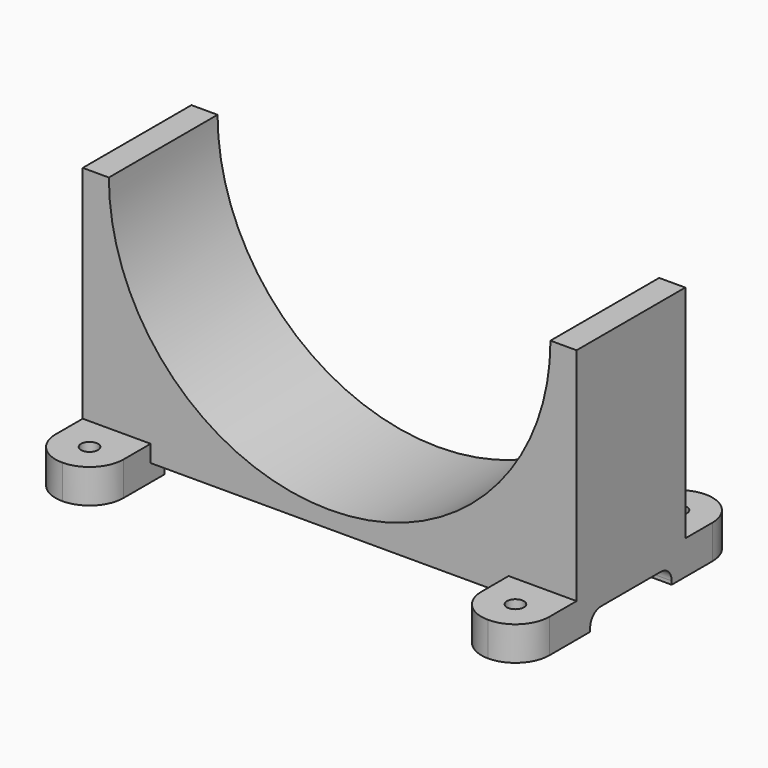
from build123d import *

# Parameters (mm, degrees)
F1_DEPTH      = 25.4
F2_W          = 12.7
F2_H          = 6.35
F3_DEPTH      = 12.7
F3_DEPTH_BACK = 38.1
F4_R          = 6.34999
F5_W          = 19.05
F5_H          = 3.175
F6_DEPTH      = 92.3136190901
F7_W          = 66.9126190901
F7_H          = 3.175
F8_DEPTH      = 38.101
F9_R          = 2.54
F10_R         = 1.5875
F11_DEPTH     = 6.351


# Not quite as in the source:
# - a fillet or chamfer is up to 0.001 mm smaller than in the source, because OpenCascade refuses the exact size


with BuildPart() as f1:
    # F0 (on Front) → F1 (new body)
    with BuildSketch(Plane.XZ):
        with BuildLine():
            ThreePointArc((41.275, 0), (0, -41.275), (-41.275, 0))
            Line((-41.275, 0), (-46.156309545, 0))
            Line((-46.156309545, 0), (-46.156309545, -47.625))
            Line((-46.156309545, -47.625), (46.156309545, -47.625))
            Line((46.156309545, -47.625), (46.156309545, 0))
            Line((46.156309545, 0), (41.275, 0))
        make_face()
    extrude(amount=F1_DEPTH)

    # F2 (on face) → F3 (join, two sides)
    with BuildSketch(Plane.XZ.offset(25.4)) as f3_sk:
        with Locations((-39.806309545, -44.45)):
            Rectangle(F2_W, F2_H)
        with Locations((39.806309545, -44.45)):
            Rectangle(F2_W, F2_H)
    extrude(amount=F3_DEPTH)
    extrude(f3_sk.sketch, amount=-F3_DEPTH_BACK)

    # F4 (radius 6.35 in the source; OpenCascade refuses exactly that, so slightly less here)
    f4_edges = [f1.edges().sort_by_distance(p)[0] for p in [
        (-46.15631, 12.7, -44.45),
        (-33.45631, 12.7, -44.45),
        (-46.15631, -38.1, -44.45),
        (-33.45631, -38.1, -44.45),
        (33.45631, -38.1, -44.45),
        (46.15631, -38.1, -44.45),
        (33.45631, 12.7, -44.45),
        (46.15631, 12.7, -44.45),
    ]]
    fillet(f4_edges, radius=F4_R)

    # F5 (on face) → F6 (cut, through all)
    with BuildSketch(Plane(origin=(-46.156309545, 0, 0), x_dir=(0, -1, 0), z_dir=(-1, 0, 0))):
        with Locations((12.7, -46.0375)):
            Rectangle(F5_W, F5_H)
    extrude(amount=-F6_DEPTH, mode=Mode.SUBTRACT)

    # F7 (on face) → F8 (cut, through all)
    with BuildSketch(Plane.XZ.offset(25.4)):
        with Locations((0, -46.0375)):
            Rectangle(F7_W, F7_H)
    extrude(amount=-F8_DEPTH, mode=Mode.SUBTRACT)

    # F9
    f9_edges = [f1.edges().sort_by_distance(p)[0] for p in [
        (-39.80631, -22.225, -44.45),
        (-39.80631, -3.175, -44.45),
        (39.80631, -3.175, -44.45),
        (39.80631, -22.225, -44.45),
    ]]
    fillet(f9_edges, radius=F9_R)

    # F10 (on face) → F11 (cut, through all)
    with BuildSketch(Plane.XY.offset(-41.275)):
        with Locations((-39.806309545, -31.75)):
            Circle(F10_R)
        with Locations((-39.806309545, 6.35)):
            Circle(F10_R)
        with Locations((39.806309545, -31.75)):
            Circle(F10_R)
        with Locations((39.806309545, 6.35)):
            Circle(F10_R)
    extrude(amount=-F11_DEPTH, mode=Mode.SUBTRACT)


solid = f1.part
